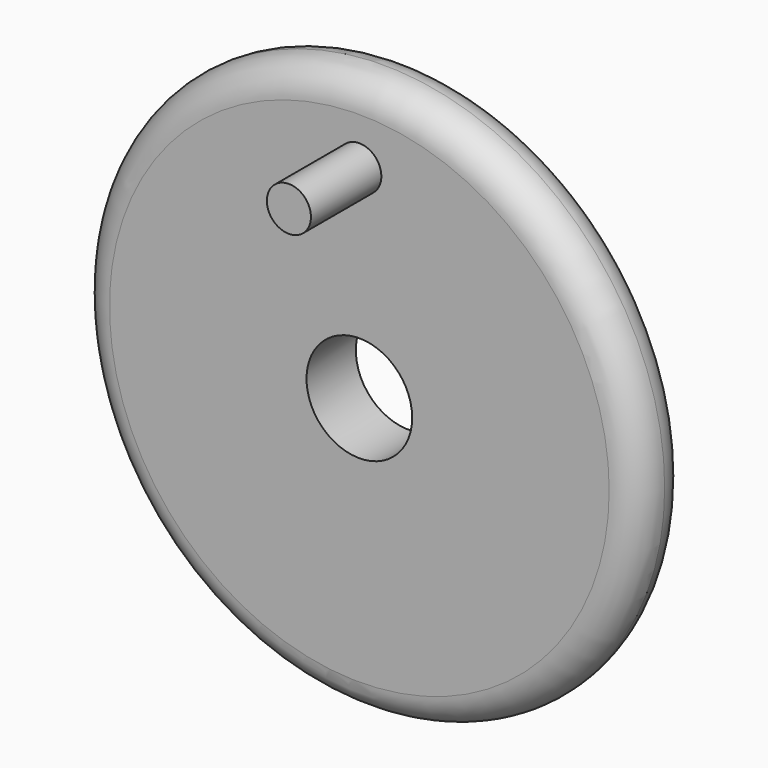
from build123d import *

# Parameters (mm, degrees)
F0_R     = 3.1875
F1_DEPTH = 0.7
F2_R     = 0.6
F3_DEPTH = 25
F4_R     = 0.34999
F5_R     = 0.25
F6_DEPTH = 1


# Not quite as in the source:
# - a fillet or chamfer is up to 0.001 mm smaller than in the source, because OpenCascade refuses the exact size


with BuildPart() as f1:
    # F0 (on Front) → F1 (new body)
    with BuildSketch(Plane.XZ):
        Circle(F0_R)
    extrude(amount=F1_DEPTH)

    # F2 (on face) → F3 (cut)
    with BuildSketch(Plane.XZ.offset(0.7)):
        Circle(F2_R)
    extrude(amount=-F3_DEPTH, mode=Mode.SUBTRACT)

    # F4 (radius 0.35 in the source; OpenCascade refuses exactly that, so slightly less here)
    f4_edges = [f1.edges().sort_by_distance(p)[0] for p in [
        (3.1875, -0.35, 0),
        (-3.1875, 0, 0),
        (-3.1875, -0.7, 0),
    ]]
    fillet(f4_edges, radius=F4_R)

    # F5 (on face) → F6 (join)
    with BuildSketch(Plane.XZ.offset(0.7)):
        with Locations((0, 2.2993473568)):
            Circle(F5_R)
    extrude(amount=F6_DEPTH)


solid = f1.part
